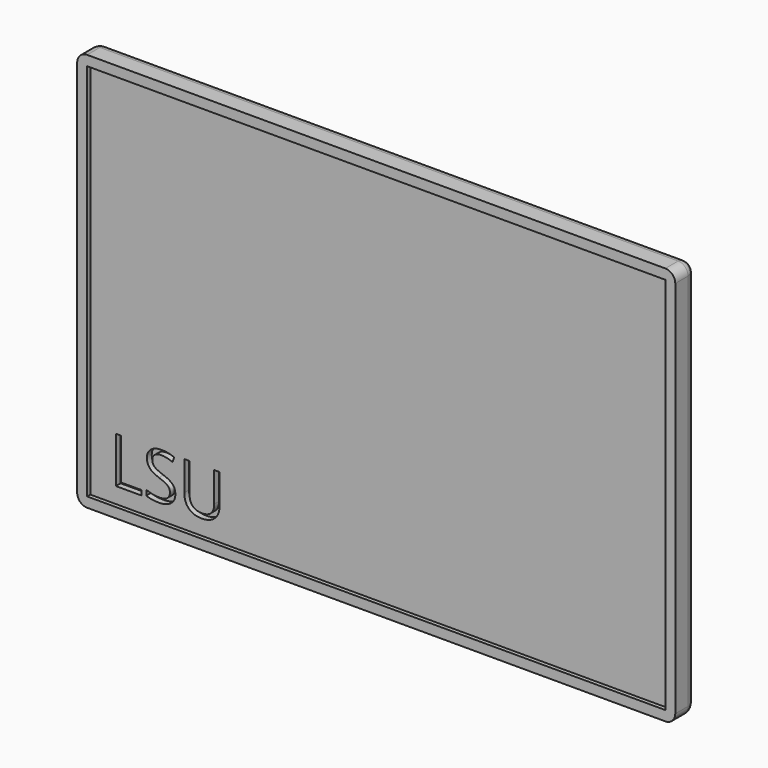
from build123d import *

# Parameters (mm, degrees)
F0_W         = 300
F0_H         = 200
F1_DEPTH     = 6.5
F2_W         = 289.9999916553
F2_H         = 189.9999916553
F3_DEPTH     = 2
F4_TEXT_SIZE = 32.3708169162
F5_DEPTH     = 5
F6_W         = 50
F6_H         = 40
F7_DEPTH     = 10
F8_R         = 9
F9_DEPTH     = 11
F10_R        = 2
F11_R        = 5


# Not quite as in the source:
# - Text() gives the source's letters only with a copy of the font that has no kerning and outlines rounded to 1/6400 em; it was checked with that copy


with BuildPart() as f1:
    # F0 (on Front) → F1 (new body, symmetric)
    with BuildSketch(Plane.XZ):
        Rectangle(F0_W, F0_H)
    extrude(amount=F1_DEPTH, both=True)

    # F2 (on face) → F3 (cut)
    with BuildSketch(Plane.XZ.offset(6.5)):
        Rectangle(F2_W, F2_H)
    extrude(amount=-F3_DEPTH, mode=Mode.SUBTRACT)

    # F4 (on face) → F5 (cut)
    with BuildSketch(Plane.XZ.offset(6.5)):
        with Locations((-135.3861838579, -87.058454752)):
            Text('LSU', F4_TEXT_SIZE, font='Open Sans', text_align=(TextAlign.LEFT, TextAlign.BOTTOM))
    extrude(amount=-F5_DEPTH, mode=Mode.SUBTRACT)

    # F6 (on face) → F7 (join)
    with BuildSketch(Plane(origin=(0, 6.5, 0), x_dir=(-1, 0, 0), z_dir=(0, 1, 0))):
        Rectangle(F6_W, F6_H)
    extrude(amount=F7_DEPTH)

    # F8 (on face) → F9 (join)
    with BuildSketch(Plane(origin=(0, 16.5, 0), x_dir=(-1, 0, 0), z_dir=(0, 1, 0))):
        Circle(F8_R)
    extrude(amount=F9_DEPTH)

    # F10
    f10_edges = [f1.edges().sort_by_distance(p)[0] for p in [
        (25, 6.5, 0),
        (0, 6.5, 20),
        (0, 6.5, -20),
        (-25, 6.5, 0),
        (-25, 16.5, 0),
        (0, 16.5, -20),
        (25, 16.5, 0),
        (0, 16.5, 20),
    ]]
    fillet(f10_edges, radius=F10_R)

    # F11
    f11_edges = [f1.edges().sort_by_distance(p)[0] for p in [
        (27, 6.5, 0),
        (0, 6.5, 22),
        (0, 6.5, -22),
        (-27, 6.5, 0),
        (0, 6.5, 100),
        (150, 6.5, 0),
        (-150, 6.5, 0),
        (0, 6.5, -100),
        (-150, 0, -100),
        (-150, 0, 100),
        (150, 0, 100),
        (150, 0, -100),
    ]]
    fillet(f11_edges, radius=F11_R)


solid = f1.part
